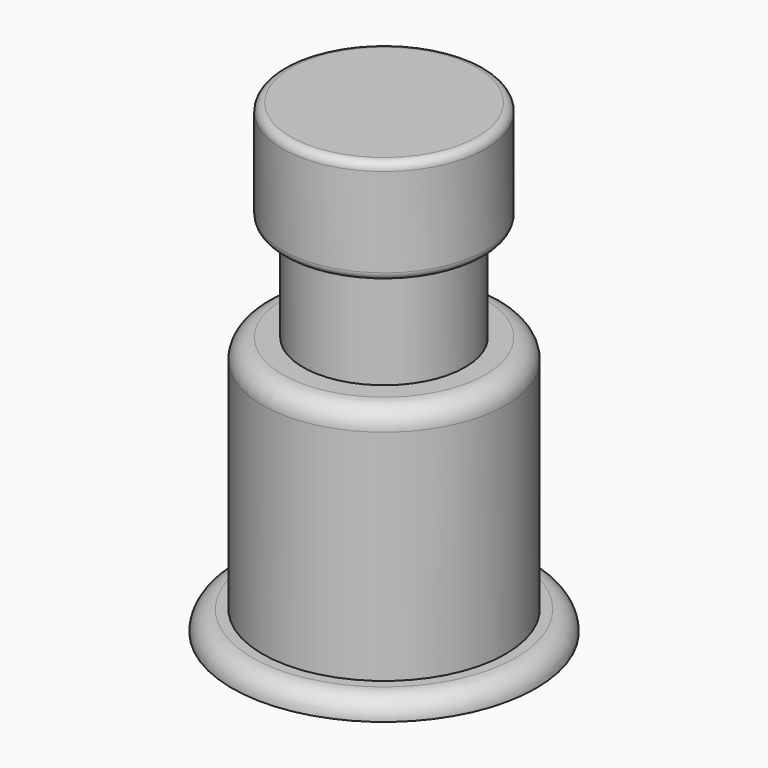
from build123d import *

# Parameters (mm, degrees)
F0_R     = 4
F1_DEPTH = 17.8
F2_R     = 5
F2_R_2   = 4
F3_DEPTH = 5.2
F4_R     = 0.4
F5_R     = 6
F5_R_2   = 4
F6_DEPTH = 12.8
F7_R     = 7.5
F7_R_2   = 6
F8_DEPTH = 1
F9_R     = 0.99999
F10_R    = 1


# Not quite as in the source:
# - a fillet or chamfer is up to 0.001 mm smaller than in the source, because OpenCascade refuses the exact size


with BuildPart() as f1:
    # F0 (on Top) → F1 (new body)
    with BuildSketch(Plane.XY):
        Circle(F0_R)
    extrude(amount=F1_DEPTH)

    # F2 (on face) → F3 (join)
    with BuildSketch(Plane.XY.offset(17.8)):
        Circle(F2_R)
        Circle(F2_R_2, mode=Mode.SUBTRACT)
        Circle(F2_R_2)
    extrude(amount=F3_DEPTH)

    # F4
    f4_edges = [f1.edges().sort_by_distance(p)[0] for p in [
        (-5, 0, 23),
        (-5, 0, 17.8),
    ]]
    fillet(f4_edges, radius=F4_R)


with BuildPart() as f6:
    # F5 (on face) → F6 (new body)
    with BuildSketch(Plane(origin=(0, 0, 0), x_dir=(1, 0, 0), z_dir=(0, 0, -1))):
        Circle(F5_R)
        Circle(F5_R_2, mode=Mode.SUBTRACT)
    extrude(amount=-F6_DEPTH)

    # F10
    f10_edges = [f6.edges().sort_by_distance(p)[0] for p in [
        (-6, 0, 12.8),
    ]]
    fillet(f10_edges, radius=F10_R)


with BuildPart() as f8:
    # F7 (on face) → F8 (new body)
    with BuildSketch(Plane(origin=(0, 0, 0), x_dir=(1, 0, 0), z_dir=(0, 0, -1))):
        Circle(F7_R)
        Circle(F7_R_2, mode=Mode.SUBTRACT)
    extrude(amount=-F8_DEPTH)

    # F9 (radius 1 in the source; OpenCascade refuses exactly that, so slightly less here)
    f9_edges = [f8.edges().sort_by_distance(p)[0] for p in [
        (-7.5, 0, 1),
    ]]
    fillet(f9_edges, radius=F9_R)


solid = Compound([f1.part, f6.part, f8.part])
